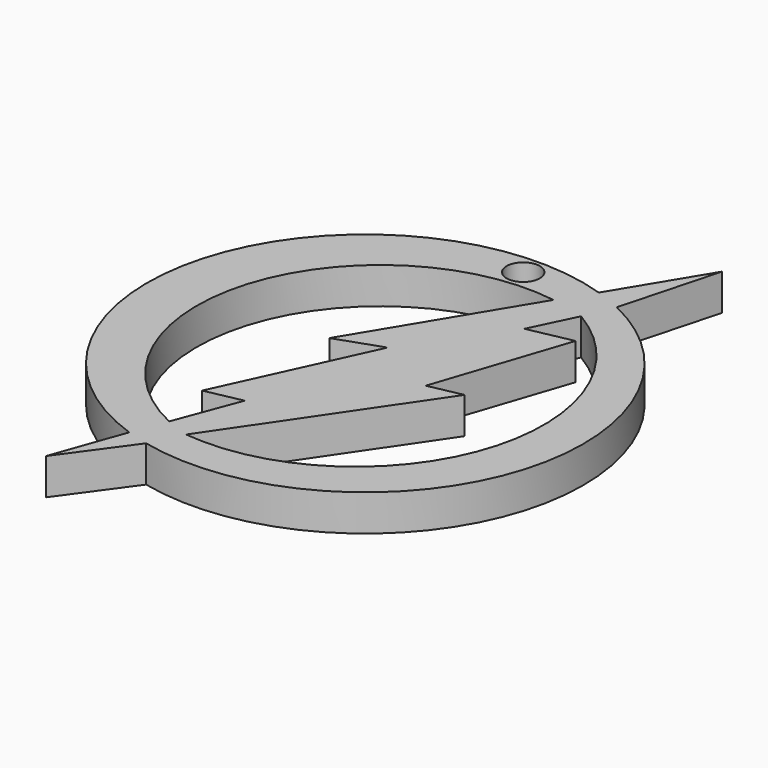
from build123d import *

# Parameters (mm, degrees)
F1_DEPTH = 6.35
F2_R     = 2.9021462782
F3_DEPTH = 12.7


# Not quite as in the source:
# - a feature names something its author has since deleted; it is built from what else it names


with BuildPart() as f1:
    # F0 (on Top) → F1 (new body)
    with BuildSketch(Plane.XY):
        with BuildLine():
            Line((16.4344385917, 34.3732341826), (21.0574541174, 51.5500892249))
            Line((21.0574541174, 51.5500892249), (11.8116865515, 36.2228389391))
            ThreePointArc((11.8116865515, 36.2228389391), (-36.1240313077, 12.1105062684), (-12.4084995786, -36.0227586146))
            Line((-12.4084995786, -36.0227586146), (-16.8951376196, -48.5777822575))
            Line((-16.8951376196, -48.5777822575), (-8.5923329011, -37.1184834727))
            ThreePointArc((-8.5923329011, -37.1184834727), (35.960270838, -12.5884439569), (16.4344385917, 34.3732341826))
        make_face()
        with BuildLine():
            Line((-5.9558603501, -18.8854594723), (-10.1813612864, -30.1025640222))
            ThreePointArc((-10.1813612864, -30.1025640222), (-27.192206018, 8.287747581), (8.3393088452, 30.6639920157))
            Line((8.3393088452, 30.6639920157), (-8.4871153459, 2.7698433524))
            Line((-8.4871153459, 2.7698433524), (-0.5399501962, 5.5430036832))
            Line((-0.5399501962, 5.5430036832), (-12.3529230131, -20.1834143903))
            Line((-12.3529230131, -20.1834143903), (-5.9558603501, -18.8854594723))
        make_face(mode=Mode.SUBTRACT)
        with BuildLine():
            Line((10.5646807305, 0), (18.2668235735, 23.0856431528))
            Line((18.2668235735, 23.0856431528), (10.5646807305, 21.522889322))
            Line((10.5646807305, 21.522889322), (14.302094467, 29.2579978704))
            ThreePointArc((14.302094467, 29.2579978704), (28.7040765344, -9.3712062036), (-5.9558603501, -31.6943168745))
            Line((-5.9558603501, -31.6943168745), (16.3907865629, 1.182108589))
            Line((16.3907865629, 1.182108589), (10.5646807305, 0))
        make_face(mode=Mode.SUBTRACT)
    extrude(amount=F1_DEPTH)

    # F2 (on face) → F3 (cut)
    with BuildSketch(Plane.XY.offset(6.35)):
        with Locations((0, 34.4884768128)):
            Circle(F2_R)
    extrude(amount=-F3_DEPTH, mode=Mode.SUBTRACT)


solid = f1.part
